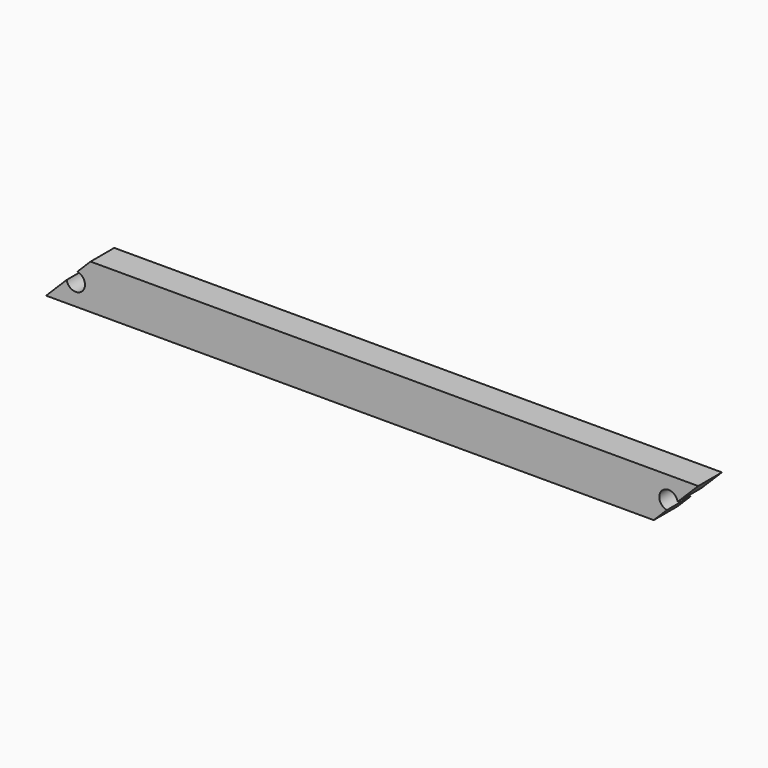
from build123d import *

# Parameters (mm, degrees)
F0_W     = 558.8
F0_H     = 38.1
F1_DEPTH = 25.4
F3_D     = 15.875
F5_DEPTH = 50.8
F7_DEPTH = 50.8


# Not quite as in the source:
# - a feature names something its author has since deleted; it is built from what else it names


with BuildPart() as f1:
    # F0 (on Front) → F1 (new body)
    with BuildSketch(Plane.XZ):
        with Locations((279.4, 19.05)):
            Rectangle(F0_W, F0_H)
    extrude(amount=F1_DEPTH)

    # F3 (through all)
    with Locations(Plane.XZ.offset(25.4)):
        with Locations((25.4, 19.05), (533.4, 19.05)):
            Hole(F3_D / 2)

    # F4 (on face) → F5 (cut)
    with BuildSketch(Plane.XZ.offset(25.4)):
        with BuildLine():
            Line((0, 38.1), (0, 0))
            Line((0, 0), (17.5966819335, 17.5966819335))
            ThreePointArc((17.5966819335, 17.5966819335), (19.7873399243, 24.6626600757), (26.8533180665, 26.8533180665))
            Line((26.8533180665, 26.8533180665), (38.1, 38.1))
            Line((38.1, 38.1), (0, 38.1))
        make_face()
    extrude(amount=-F5_DEPTH, mode=Mode.SUBTRACT)

    # F6 (on face) → F7 (cut)
    with BuildSketch(Plane.XZ.offset(25.4)):
        with BuildLine():
            Line((558.8, 0), (558.8, 38.1))
            Line((558.8, 38.1), (541.2033180665, 20.5033180665))
            ThreePointArc((541.2033180665, 20.5033180665), (541.3038833305, 19.7797496478), (541.3375, 19.05))
            ThreePointArc((541.3375, 19.05), (538.4728785762, 12.9450995748), (531.9466819335, 11.2466819335))
            Line((531.9466819335, 11.2466819335), (520.7, 0))
            Line((520.7, 0), (558.8, 0))
        make_face()
    extrude(amount=-F7_DEPTH, mode=Mode.SUBTRACT)


solid = f1.part
